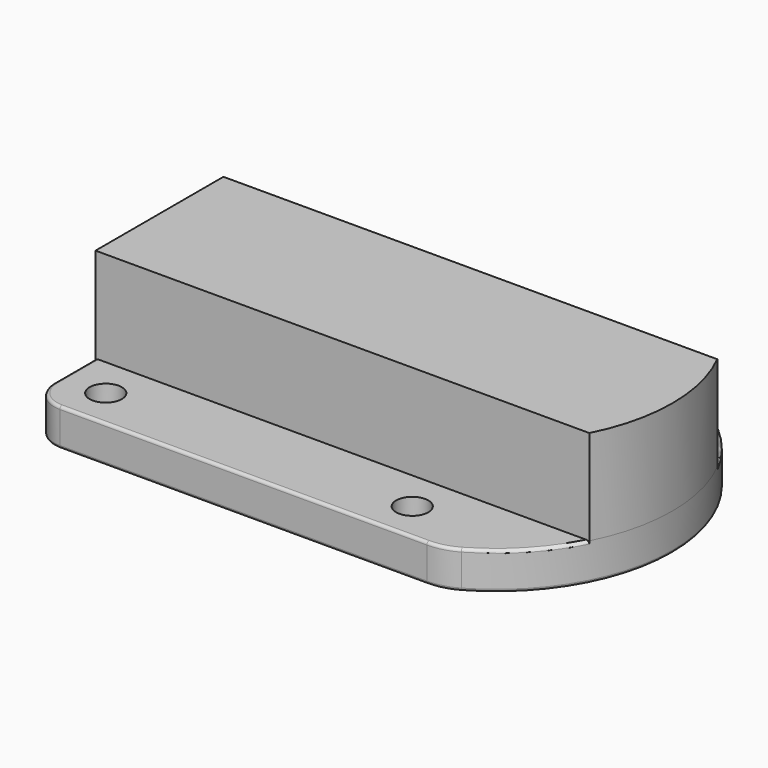
from build123d import *

# Parameters (mm, degrees)
F0_R         = 2.8
F1_DEPTH     = 6.5
F3_DEPTH     = 16.5
F4_T1_DEPTH  = 63.8184719387
F4_T3_DEPTH  = 45.8
F4_T5_DEPTH  = 9
F4_T7_DEPTH  = 9
F4_T10_ANGLE = 90
F4_T12_ANGLE = 120.4504110916
F4_T14_ANGLE = 90
F4_T16_ANGLE = 90
F4_T18_ANGLE = 29.7747944542
F4_T20_ANGLE = 29.7747944542
F4_T22_ANGLE = 29.7747944542
F4_T26_ANGLE = 35.5690080159
F4_T29_ANGLE = 90
F4_T33_ANGLE = 35.5690080159
F4_T36_ANGLE = 29.7747944542
F5_SIZE      = 1.56


# Not quite as in the source:
# - a fillet or chamfer that OpenCascade refuses, or shapes differently, is made with other operations: its cross-section is extruded or revolved along the edge and cut away or added


with BuildPart() as f1:
    # F0 (on Top) → F1 (new body)
    with BuildSketch(Plane.XY):
        with BuildLine():
            Line((-38.8770699501, 16.9000072956), (-38.8770699501, -28.8999927044))
            ThreePointArc((-38.8770699501, -28.8999927044), (-37.412603856, -32.4355266103), (-33.8770699501, -33.8999927044))
            Line((-33.8770699501, -33.8999927044), (29.9414019886, -33.8999927044))
            ThreePointArc((29.9414019886, -33.8999927044), (32.5106042183, -33.5643188528), (34.9073236464, -32.579832685))
            ThreePointArc((34.9073236464, -32.579832685), (50.3229300499, -5.9999927044), (34.9073236464, 20.5798472762))
            ThreePointArc((34.9073236464, 20.5798472762), (32.5106042183, 21.564333444), (29.9414019886, 21.9000072956))
            Line((29.9414019886, 21.9000072956), (-33.8770699501, 21.9000072956))
            ThreePointArc((-33.8770699501, 21.9000072956), (-37.412603856, 20.4355412015), (-38.8770699501, 16.9000072956))
        make_face()
        with Locations((-31.4170904458, -26.9999932498)):
            Circle(F0_R, mode=Mode.SUBTRACT)
        with Locations((21.8729300499, -26.9999927044)):
            Circle(F0_R, mode=Mode.SUBTRACT)
        with Locations((-31.4170904458, 15.0000071153)):
            Circle(F0_R, mode=Mode.SUBTRACT)
        with Locations((21.8729300499, 15.0000072956)):
            Circle(F0_R, mode=Mode.SUBTRACT)
    extrude(amount=F1_DEPTH)

    # F2 (on face) → F3 (join)
    with BuildSketch(Plane.XY.offset(6.5)):
        with BuildLine():
            Line((-38.8770699501, 7.9000072956), (-38.8770699501, -5.9999927044))
            Line((-38.8770699501, -5.9999927044), (-38.8770699501, -19.8999927044))
            Line((-38.8770699501, -19.8999927044), (46.9864613892, -19.8999927044))
            ThreePointArc((46.9864613892, -19.8999927044), (50.3229300499, -5.9999927044), (46.9864613892, 7.9000072956))
            Line((46.9864613892, 7.9000072956), (-38.8770699501, 7.9000072956))
        make_face()
    extrude(amount=F3_DEPTH)

    # F4: fillet of radius 0.5 on 18 edges, made by hand

    # F4_s2 → F4_t1 (cut)
    with BuildSketch(Plane.YZ.offset(-33.8770699501)):
        with BuildLine():
            ThreePointArc((21.9000072956, 0.5), (21.7535606862, 0.1464466094), (21.4000072956, 0))
            Line((21.4000072956, 0), (21.9000072956, 0))
            Line((21.9000072956, 0), (21.9000072956, 0.5))
        make_face()
        with BuildLine():
            ThreePointArc((21.9000072956, 6), (21.7535606862, 6.3535533906), (21.4000072956, 6.5))
            Line((21.4000072956, 6.5), (21.9000072956, 6.5))
            Line((21.9000072956, 6.5), (21.9000072956, 6))
        make_face()
        with BuildLine():
            ThreePointArc((-33.3999927044, 6.5), (-33.753546095, 6.3535533906), (-33.8999927044, 6))
            Line((-33.8999927044, 6), (-33.8999927044, 6.5))
            Line((-33.8999927044, 6.5), (-33.3999927044, 6.5))
        make_face()
        with BuildLine():
            ThreePointArc((-33.3999927044, 0), (-33.753546095, 0.1464466094), (-33.8999927044, 0.5))
            Line((-33.8999927044, 0.5), (-33.8999927044, 0))
            Line((-33.8999927044, 0), (-33.3999927044, 0))
        make_face()
    extrude(amount=F4_T1_DEPTH, mode=Mode.SUBTRACT)

    # F4_s4 → F4_t3 (cut)
    with BuildSketch(Plane.XZ.offset(-16.9000072956)):
        with BuildLine():
            ThreePointArc((-38.8770699501, 0.5), (-38.7306233407, 0.1464466094), (-38.3770699501, 0))
            Line((-38.3770699501, 0), (-38.8770699501, 0))
            Line((-38.8770699501, 0), (-38.8770699501, 0.5))
        make_face()
    extrude(amount=F4_T3_DEPTH, mode=Mode.SUBTRACT)

    # F4_s6 → F4_t5 (cut)
    with BuildSketch(Plane.XZ.offset(-16.9000072956)):
        with BuildLine():
            ThreePointArc((-38.8770699501, 6), (-38.7306233407, 6.3535533906), (-38.3770699501, 6.5))
            Line((-38.3770699501, 6.5), (-38.8770699501, 6.5))
            Line((-38.8770699501, 6.5), (-38.8770699501, 6))
        make_face()
    extrude(amount=F4_T5_DEPTH, mode=Mode.SUBTRACT)

    # F4_s8 → F4_t7 (cut)
    with BuildSketch(Plane.XZ.offset(19.8999927044)):
        with BuildLine():
            ThreePointArc((-38.8770699501, 6), (-38.7306233407, 6.3535533906), (-38.3770699501, 6.5))
            Line((-38.3770699501, 6.5), (-38.8770699501, 6.5))
            Line((-38.8770699501, 6.5), (-38.8770699501, 6))
        make_face()
    extrude(amount=F4_T7_DEPTH, mode=Mode.SUBTRACT)

    # F4_s9 → F4_t10 (revolve, cut)
    with BuildSketch(Plane.YZ.offset(-33.8770699501)):
        with BuildLine():
            ThreePointArc((21.9000072956, 0.5), (21.7535606862, 0.1464466094), (21.4000072956, 0))
            Line((21.4000072956, 0), (21.9000072956, 0))
            Line((21.9000072956, 0), (21.9000072956, 0.5))
        make_face()
    revolve(axis=Axis((-33.8770699501, 16.9000072956, 0), (0, 0, 1)), revolution_arc=F4_T10_ANGLE, mode=Mode.SUBTRACT)

    # F4_s11 → F4_t12 (revolve, cut)
    with BuildSketch(Plane(origin=(12.2560283734, 7.0119353437, 0), x_dir=(0, 0, 1), z_dir=(-0.8679839981, -0.4965921658, 0))):
        with BuildLine():
            ThreePointArc((0, -45.1134768811), (0.1464466094, -45.4670302717), (0.5, -45.6134768811))
            Line((0.5, -45.6134768811), (0, -45.6134768811))
            Line((0, -45.6134768811), (0, -45.1134768811))
        make_face()
    revolve(axis=Axis((19.7004300499, -5.9999927044, 0), (0, 0, 1)), revolution_arc=F4_T12_ANGLE, mode=Mode.SUBTRACT)

    # F4_s13 → F4_t14 (revolve, cut)
    with BuildSketch(Plane.YZ.offset(-33.8770699501)):
        with BuildLine():
            ThreePointArc((21.9000072956, 6), (21.7535606862, 6.3535533906), (21.4000072956, 6.5))
            Line((21.4000072956, 6.5), (21.9000072956, 6.5))
            Line((21.9000072956, 6.5), (21.9000072956, 6))
        make_face()
    revolve(axis=Axis((-33.8770699501, 16.9000072956, 6.5), (0, 0, 1)), revolution_arc=F4_T14_ANGLE, mode=Mode.SUBTRACT)

    # F4_s15 → F4_t16 (revolve, cut)
    with BuildSketch(Plane.XZ.offset(28.8999927044)):
        with BuildLine():
            ThreePointArc((-38.3770699501, 0), (-38.7306233407, 0.1464466094), (-38.8770699501, 0.5))
            Line((-38.8770699501, 0.5), (-38.8770699501, 0))
            Line((-38.8770699501, 0), (-38.3770699501, 0))
        make_face()
    revolve(axis=Axis((-33.8770699501, -28.8999927044, 0), (0, 0, 1)), revolution_arc=F4_T16_ANGLE, mode=Mode.SUBTRACT)

    # F4_s17 → F4_t18 (revolve, cut)
    with BuildSketch(Plane.YZ.offset(29.9414019886)):
        with BuildLine():
            ThreePointArc((-33.3999927044, 0), (-33.753546095, 0.1464466094), (-33.8999927044, 0.5))
            Line((-33.8999927044, 0.5), (-33.8999927044, 0))
            Line((-33.8999927044, 0), (-33.3999927044, 0))
        make_face()
    revolve(axis=Axis((29.9414019886, -23.8999927044, 0), (0, 0, 1)), revolution_arc=F4_T18_ANGLE, mode=Mode.SUBTRACT)

    # F4_s19 → F4_t20 (revolve, cut)
    with BuildSketch(Plane(origin=(17.4284307256, -9.9711770948, 0), x_dir=(0, 0, 1), z_dir=(0.8679839981, -0.4965921658, 0))):
        with BuildLine():
            ThreePointArc((0, -34.6976815693), (0.1464466094, -35.0512349599), (0.5, -35.1976815693))
            Line((0.5, -35.1976815693), (0, -35.1976815693))
            Line((0, -35.1976815693), (0, -34.6976815693))
        make_face()
    revolve(axis=Axis((29.9414019886, 11.9000072956, 0), (0, 0, 1)), revolution_arc=F4_T20_ANGLE, mode=Mode.SUBTRACT)

    # F4_s21 → F4_t22 (revolve, cut)
    with BuildSketch(Plane(origin=(17.4284307256, -9.9711770948, 0), x_dir=(0, 0, 1), z_dir=(0.8679839981, -0.4965921658, 0))):
        with BuildLine():
            ThreePointArc((6.5, -34.6976815693), (6.3535533906, -35.0512349599), (6, -35.1976815693))
            Line((6, -35.1976815693), (6.5, -35.1976815693))
            Line((6.5, -35.1976815693), (6.5, -34.6976815693))
        make_face()
    revolve(axis=Axis((29.9414019886, 11.9000072956, 6.5), (0, 0, 1)), revolution_arc=F4_T22_ANGLE, mode=Mode.SUBTRACT)


with BuildPart() as f4_tool24:
    # F4_s25 → F4_t26 (revolve)
    with BuildSketch(Plane(origin=(5.7033446243, -12.4249727464, 0), x_dir=(0, 0, 1), z_dir=(0.4171723997, -0.9088273703, 0))):
        with BuildLine():
            ThreePointArc((6.5, -45.5237586807), (6.3535533906, -45.8773120713), (6, -46.0237586807))
            Line((6, -46.0237586807), (6.5, -46.0237586807))
            Line((6.5, -46.0237586807), (6.5, -45.5237586807))
        make_face()
    revolve(axis=Axis((19.7004300499, -5.9999927044, 6.5), (0, 0, 1)), revolution_arc=F4_T26_ANGLE)

    split(bisect_by=Plane.XZ.offset(-7.9000072956), keep=Keep.BOTTOM)


with BuildPart() as f1_1:
    add(f1.part)

    # F4_t23: cut F4_tool24
    add(f4_tool24.part, mode=Mode.SUBTRACT)

    # F4_s28 → F4_t29 (revolve, cut)
    with BuildSketch(Plane.XZ.offset(28.8999927044)):
        with BuildLine():
            ThreePointArc((-38.8770699501, 6), (-38.7306233407, 6.3535533906), (-38.3770699501, 6.5))
            Line((-38.3770699501, 6.5), (-38.8770699501, 6.5))
            Line((-38.8770699501, 6.5), (-38.8770699501, 6))
        make_face()
    revolve(axis=Axis((-33.8770699501, -28.8999927044, 6.5), (0, 0, 1)), revolution_arc=F4_T29_ANGLE, mode=Mode.SUBTRACT)


with BuildPart() as f4_tool31:
    # F4_s32 → F4_t33 (revolve)
    with BuildSketch(Plane(origin=(12.2560283734, 7.0119353437, 0), x_dir=(0, 0, 1), z_dir=(-0.8679839981, -0.4965921658, 0))):
        with BuildLine():
            ThreePointArc((6.5, -45.1134768811), (6.3535533906, -45.4670302717), (6, -45.6134768811))
            Line((6, -45.6134768811), (6.5, -45.6134768811))
            Line((6.5, -45.6134768811), (6.5, -45.1134768811))
        make_face()
    revolve(axis=Axis((19.7004300499, -5.9999927044, 6.5), (0, 0, 1)), revolution_arc=F4_T33_ANGLE)

    split(bisect_by=Plane.XZ.offset(19.8999927044), keep=Keep.TOP)


with BuildPart() as f1_2:
    add(f1_1.part)

    # F4_t30: cut F4_tool31
    add(f4_tool31.part, mode=Mode.SUBTRACT)

    # F4_s35 → F4_t36 (revolve, cut)
    with BuildSketch(Plane.YZ.offset(29.9414019886)):
        with BuildLine():
            ThreePointArc((-33.3999927044, 6.5), (-33.753546095, 6.3535533906), (-33.8999927044, 6))
            Line((-33.8999927044, 6), (-33.8999927044, 6.5))
            Line((-33.8999927044, 6.5), (-33.3999927044, 6.5))
        make_face()
    revolve(axis=Axis((29.9414019886, -23.8999927044, 6.5), (0, 0, 1)), revolution_arc=F4_T36_ANGLE, mode=Mode.SUBTRACT)

    # F5
    f5_edges = [f1_2.edges().sort_by_distance(p)[0] for p in [
        (-34.21709, 15.000007, 0),
        (-34.21709, -26.999993, 0),
        (19.07293, -26.999993, 0),
        (19.07293, 15.000007, 0),
    ]]
    chamfer(f5_edges, length=F5_SIZE)


solid = f1_2.part
